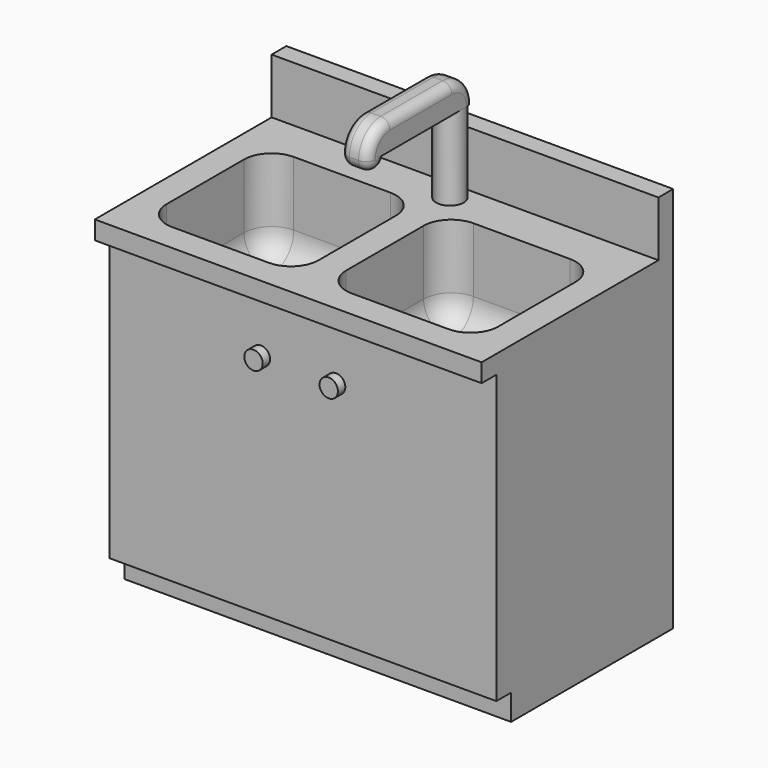
from build123d import *

# Parameters (mm, degrees)
F0_W          = 1066.8
F0_H          = 609.6
F1_DEPTH      = 914.4
F2_W          = 1066.8
F2_H          = 50.8
F2_H_2        = 609.6
F3_DEPTH      = 50.8
F4_W          = 1066.8
F4_H          = 50.8
F5_DEPTH      = 152.4
F4_W_2        = 419.1
F4_H_2        = 419.1
F6_DEPTH      = 254
F7_R          = 76.2
F4_R          = 38.1
F8_DEPTH      = 228.6
F10_DEPTH     = 38.1
F11_T3_DEPTH  = 213.5462481737
F11_T6_DEPTH  = 213.5462481737
F11_T9_ANGLE  = 180
F11_T12_ANGLE = 180
F11_T15_ANGLE = 90
F11_T18_ANGLE = 90
F11_T21_ANGLE = 90
F11_T24_ANGLE = 90
F12_W         = 812.8
F12_H         = 355.6
F13_DEPTH     = 431.292
F14_W         = 1066.8
F14_H         = 71.1514726281
F15_DEPTH     = 50.8
F16_R         = 25.4
F17_DEPTH     = 25.4


# Not quite as in the source:
# - a fillet or chamfer that OpenCascade refuses, or shapes differently, is made with other operations: its cross-section is extruded or revolved along the edge and cut away or added


with BuildPart() as f1:
    # F0 (on Top) → F1 (new body)
    with BuildSketch(Plane.XY):
        Rectangle(F0_W, F0_H)
    extrude(amount=F1_DEPTH)

    # F2 (on face) → F3 (join)
    with BuildSketch(Plane.XY.offset(914.4)):
        with Locations((0, -330.2)):
            Rectangle(F2_W, F2_H)
        Rectangle(F2_W, F2_H_2)
    extrude(amount=-F3_DEPTH)

    # F4 (on face) → F5 (join)
    with BuildSketch(Plane.XY.offset(914.4)):
        with Locations((0, 279.4)):
            Rectangle(F4_W, F4_H)
    extrude(amount=F5_DEPTH)

    # F4 (on face) → F6 (cut)
    with BuildSketch(Plane.XY.offset(914.4)):
        with Locations((-247.65, -69.85)):
            Rectangle(F4_W_2, F4_H_2)
        with Locations((247.65, -69.85)):
            Rectangle(F4_W_2, F4_H_2)
    extrude(amount=-F6_DEPTH, mode=Mode.SUBTRACT)

    # F7
    f7_edges = [f1.edges().sort_by_distance(p)[0] for p in [
        (-247.65, 139.7, 660.4),
        (-457.2, -69.85, 660.4),
        (-247.65, -279.4, 660.4),
        (-38.1, -69.85, 660.4),
        (247.65, 139.7, 660.4),
        (38.1, -69.85, 660.4),
        (247.65, -279.4, 660.4),
        (457.2, -69.85, 660.4),
        (457.2, 139.7, 787.4),
        (38.1, 139.7, 787.4),
        (457.2, -279.4, 787.4),
        (38.1, -279.4, 787.4),
        (-457.2, -279.4, 787.4),
        (-38.1, -279.4, 787.4),
        (-38.1, 139.7, 787.4),
        (-457.2, 139.7, 787.4),
    ]]
    fillet(f7_edges, radius=F7_R)

    # F4 (on face) → F8 (join)
    with BuildSketch(Plane.XY.offset(914.4)):
        with Locations((0, 201.7975896597)):
            Circle(F4_R)
    extrude(amount=F8_DEPTH)

    # F9 (on Right) → F10 (join, symmetric)
    with BuildSketch(Plane.YZ):
        with BuildLine():
            Line((160.8298355818, 1219.2), (-52.7164125919, 1219.2))
            ThreePointArc((-52.7164125919, 1219.2), (-106.5979493183, 1196.8815367264), (-128.9164125919, 1143))
            ThreePointArc((-128.9164125919, 1143), (-97.7595895529, 1174.1568230391), (-66.6027665138, 1143))
            Line((-66.6027665138, 1143), (237.0298355818, 1143))
            ThreePointArc((237.0298355818, 1143), (214.7113723082, 1196.8815367264), (160.8298355818, 1219.2))
        make_face()
        with BuildLine():
            ThreePointArc((-66.6027665138, 1143), (-97.7595895529, 1174.1568230391), (-128.9164125919, 1143))
            Line((-128.9164125919, 1143), (-66.6027665138, 1143))
        make_face()
        with BuildLine():
            Line((-66.6027665138, 1143), (-128.9164125919, 1143))
            ThreePointArc((-128.9164125919, 1143), (-97.7595895529, 1111.8431769609), (-66.6027665138, 1143))
        make_face()
    extrude(amount=F10_DEPTH, both=True)

    # F11: fillet of radius 25.4 on 8 edges, made by hand


with BuildPart() as f11_tool1:
    # F11_s2 → F11_t3 (new body)
    with BuildSketch(Plane.XZ.offset(-160.8298355818)):
        with BuildLine():
            ThreePointArc((38.1, 1193.8), (30.6605122421, 1211.7605122421), (12.7, 1219.2))
            Line((12.7, 1219.2), (12.7, 1219.708))
            Line((12.7, 1219.708), (38.608, 1219.708))
            Line((38.608, 1219.708), (38.608, 1193.8))
            Line((38.608, 1193.8), (38.1, 1193.8))
        make_face()
    extrude(amount=F11_T3_DEPTH)


with BuildPart() as f11_tool4:
    # F11_s5 → F11_t6 (new body)
    with BuildSketch(Plane.XZ.offset(-160.8298355818)):
        with BuildLine():
            ThreePointArc((-38.1, 1193.8), (-30.6605122421, 1211.7605122421), (-12.7, 1219.2))
            Line((-12.7, 1219.2), (-12.7, 1219.708))
            Line((-12.7, 1219.708), (-38.608, 1219.708))
            Line((-38.608, 1219.708), (-38.608, 1193.8))
            Line((-38.608, 1193.8), (-38.1, 1193.8))
        make_face()
    extrude(amount=F11_T6_DEPTH)


with BuildPart() as f11_tool7:
    # F11_s8 → F11_t9 (revolve)
    with BuildSketch(Plane.XY.offset(1143)):
        with BuildLine():
            ThreePointArc((-12.7, -128.9164125919), (-30.6605122421, -121.4769248341), (-38.1, -103.5164125919))
            Line((-38.1, -103.5164125919), (-38.608, -103.5164125919))
            Line((-38.608, -103.5164125919), (-38.608, -129.4244125919))
            Line((-38.608, -129.4244125919), (-12.7, -129.4244125919))
            Line((-12.7, -129.4244125919), (-12.7, -128.9164125919))
        make_face()
    revolve(axis=Axis((-38.1, -97.7595895529, 1143), (1, 0, 0)), revolution_arc=F11_T9_ANGLE)


with BuildPart() as f11_tool10:
    # F11_s11 → F11_t12 (revolve)
    with BuildSketch(Plane.XY.offset(1143)):
        with BuildLine():
            ThreePointArc((12.7, -128.9164125919), (30.6605122421, -121.4769248341), (38.1, -103.5164125919))
            Line((38.1, -103.5164125919), (38.608, -103.5164125919))
            Line((38.608, -103.5164125919), (38.608, -129.4244125919))
            Line((38.608, -129.4244125919), (12.7, -129.4244125919))
            Line((12.7, -129.4244125919), (12.7, -128.9164125919))
        make_face()
    revolve(axis=Axis((38.1, -97.7595895529, 1143), (1, 0, 0)), revolution_arc=F11_T12_ANGLE)


with BuildPart() as f11_tool13:
    # F11_s14 → F11_t15 (revolve)
    with BuildSketch(Plane.XZ.offset(52.7164125919)):
        with BuildLine():
            ThreePointArc((38.1, 1193.8), (30.6605122421, 1211.7605122421), (12.7, 1219.2))
            Line((12.7, 1219.2), (12.7, 1219.708))
            Line((12.7, 1219.708), (38.608, 1219.708))
            Line((38.608, 1219.708), (38.608, 1193.8))
            Line((38.608, 1193.8), (38.1, 1193.8))
        make_face()
    revolve(axis=Axis((38.1, -52.7164125919, 1143), (1, 0, 0)), revolution_arc=F11_T15_ANGLE)


with BuildPart() as f11_tool16:
    # F11_s17 → F11_t18 (revolve)
    with BuildSketch(Plane.XY.offset(1143)):
        with BuildLine():
            ThreePointArc((38.1, 211.6298355818), (30.6605122421, 229.5903478239), (12.7, 237.0298355818))
            Line((12.7, 237.0298355818), (12.7, 237.5378355818))
            Line((12.7, 237.5378355818), (38.608, 237.5378355818))
            Line((38.608, 237.5378355818), (38.608, 211.6298355818))
            Line((38.608, 211.6298355818), (38.1, 211.6298355818))
        make_face()
    revolve(axis=Axis((38.1, 160.8298355818, 1143), (1, 0, 0)), revolution_arc=F11_T18_ANGLE)


with BuildPart() as f11_tool19:
    # F11_s20 → F11_t21 (revolve)
    with BuildSketch(Plane.XZ.offset(52.7164125919)):
        with BuildLine():
            ThreePointArc((-38.1, 1193.8), (-30.6605122421, 1211.7605122421), (-12.7, 1219.2))
            Line((-12.7, 1219.2), (-12.7, 1219.708))
            Line((-12.7, 1219.708), (-38.608, 1219.708))
            Line((-38.608, 1219.708), (-38.608, 1193.8))
            Line((-38.608, 1193.8), (-38.1, 1193.8))
        make_face()
    revolve(axis=Axis((-38.1, -52.7164125919, 1143), (1, 0, 0)), revolution_arc=F11_T21_ANGLE)


with BuildPart() as f11_tool22:
    # F11_s23 → F11_t24 (revolve)
    with BuildSketch(Plane.XY.offset(1143)):
        with BuildLine():
            ThreePointArc((-38.1, 211.6298355818), (-30.6605122421, 229.5903478239), (-12.7, 237.0298355818))
            Line((-12.7, 237.0298355818), (-12.7, 237.5378355818))
            Line((-12.7, 237.5378355818), (-38.608, 237.5378355818))
            Line((-38.608, 237.5378355818), (-38.608, 211.6298355818))
            Line((-38.608, 211.6298355818), (-38.1, 211.6298355818))
        make_face()
    revolve(axis=Axis((-38.1, 160.8298355818, 1143), (1, 0, 0)), revolution_arc=F11_T24_ANGLE)


with BuildPart() as f1_1:
    add(f1.part)

    # F11_t25: cut F11_tool1, F11_tool4, F11_tool7, F11_tool10, F11_tool13, F11_tool16, F11_tool19, F11_tool22
    add([f11_tool1.part, f11_tool4.part, f11_tool7.part, f11_tool10.part, f11_tool13.part, f11_tool16.part, f11_tool19.part, f11_tool22.part], mode=Mode.SUBTRACT)

    # F12 (on face) → F13 (cut)
    with BuildSketch(Plane(origin=(0, 0, 0), x_dir=(1, 0, 0), z_dir=(0, 0, -1))):
        Rectangle(F12_W, F12_H)
    extrude(amount=-F13_DEPTH, mode=Mode.SUBTRACT)

    # F14 (on face) → F15 (cut)
    with BuildSketch(Plane.XZ.offset(304.8)):
        with Locations((0, 35.5757363141)):
            Rectangle(F14_W, F14_H)
    extrude(amount=-F15_DEPTH, mode=Mode.SUBTRACT)

    # F16 (on face) → F17 (join)
    with BuildSketch(Plane.XZ.offset(304.8)):
        with Locations((-116.0961332864, 698.1492042542)):
            Circle(F16_R)
        with Locations((91.3885235786, 698.1492042542)):
            Circle(F16_R)
    extrude(amount=F17_DEPTH)


solid = f1_1.part
